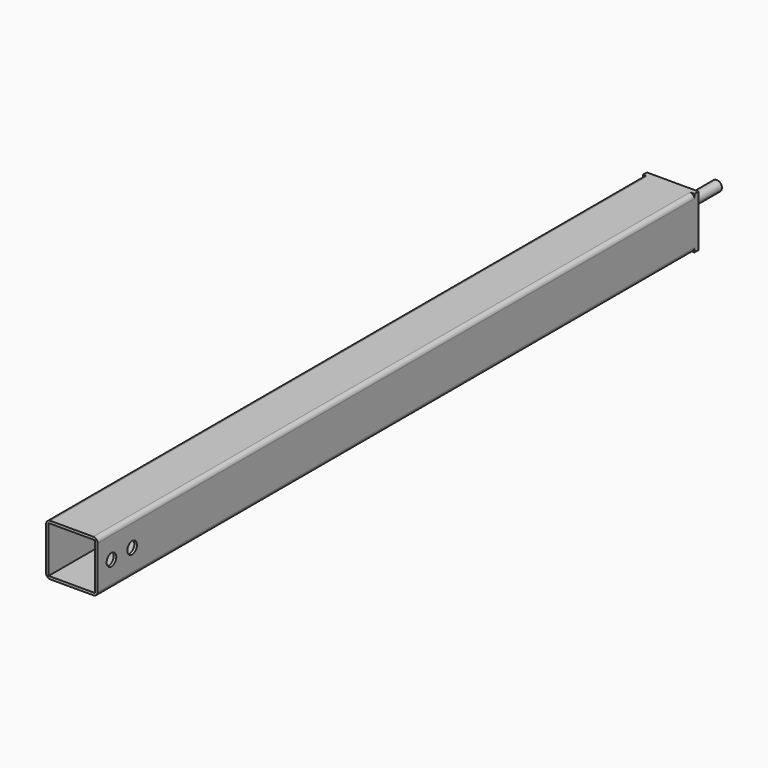
from build123d import *

# Parameters (mm, degrees)
F0_W     = 54
F0_H     = 54
F1_DEPTH = 867
F2_R     = 7
F3_DEPTH = 3
F4_W     = 60
F4_H     = 60
F4_R     = 6
F5_DEPTH = 6
F7_R     = 6
F8_DEPTH = 70


# Not quite as in the source:
# - a feature names something its author has since deleted; it is built from what else it names


with BuildPart() as f1:
    # F0 (on Front) → F1 (new body)
    with BuildSketch(Plane.XZ):
        with BuildLine():
            ThreePointArc((-28.9867345989, -60.995567819), (-30.4512006929, -57.460033913), (-33.9867345989, -55.995567819))
            Line((-33.9867345989, -55.995567819), (-83.9867345989, -55.995567819))
            ThreePointArc((-83.9867345989, -55.995567819), (-87.5222685048, -57.460033913), (-88.9867345989, -60.995567819))
            Line((-88.9867345989, -60.995567819), (-88.9867345989, -110.995567819))
            ThreePointArc((-88.9867345989, -110.995567819), (-87.5222685048, -114.5311017249), (-83.9867345989, -115.995567819))
            Line((-83.9867345989, -115.995567819), (-33.9867345989, -115.995567819))
            ThreePointArc((-33.9867345989, -115.995567819), (-30.4512006929, -114.5311017249), (-28.9867345989, -110.995567819))
            Line((-28.9867345989, -110.995567819), (-28.9867345989, -60.995567819))
        make_face()
        with Locations((-58.9867345989, -85.995567819)):
            Rectangle(F0_W, F0_H, mode=Mode.SUBTRACT)
    extrude(amount=-F1_DEPTH)

    # F2 (on face) → F3 (cut, through all)
    with BuildSketch(Plane.YZ.offset(-28.9867345989)):
        with Locations((20, -85.995567819)):
            Circle(F2_R)
        with Locations((50, -85.995567819)):
            Circle(F2_R)
    extrude(amount=-F3_DEPTH, mode=Mode.SUBTRACT)

    # F4 (on face) → F5 (join)
    with BuildSketch(Plane(origin=(0, 867, 0), x_dir=(-1, 0, 0), z_dir=(0, 1, 0))):
        with Locations((58.9867345989, -85.995567819)):
            Rectangle(F4_W, F4_H)
        with Locations((58.9867345989, -85.995567819)):
            Circle(F4_R, mode=Mode.SUBTRACT)
    extrude(amount=F5_DEPTH)

    # F7 (on offset) → F8 (join)
    with BuildSketch(Plane(origin=(0, 867, 0), x_dir=(-1, 0, 0), z_dir=(0, 1, 0))):
        with Locations((58.9867345989, -85.995567819)):
            Circle(F7_R)
    extrude(amount=F8_DEPTH)


solid = f1.part
